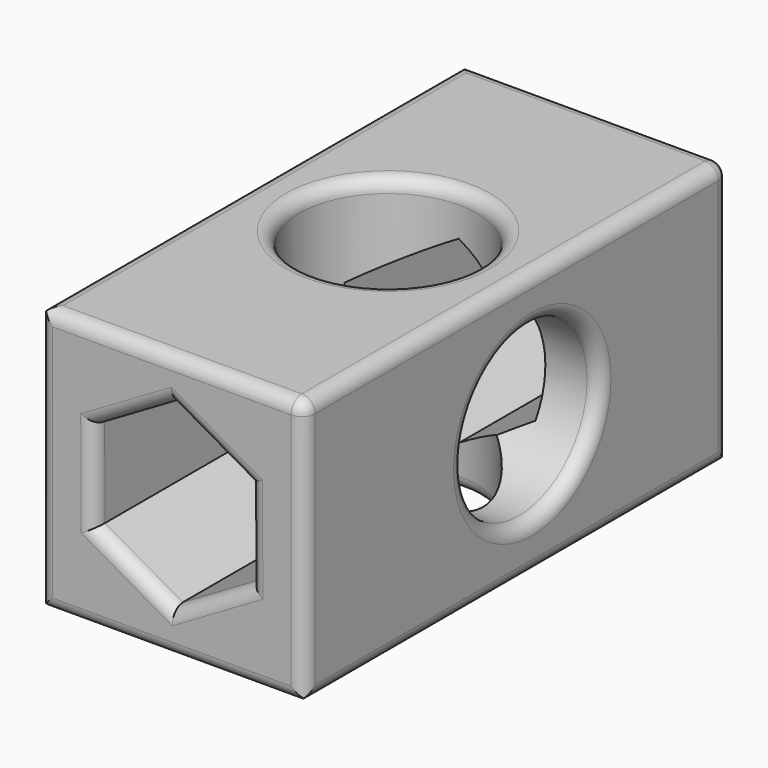
from build123d import *

# Parameters (mm, degrees)
F0_W           = 100
F0_H           = 100
F1_DEPTH       = 200
F2_DEPTH       = 25
F3_R           = 27.377441892
F4_DEPTH       = 67
F5_R           = 33.5014212571
F6_DEPTH       = 100.001
F7_R           = 32.0841158334
F8_DEPTH       = 50.001
F9_R           = 5
F10_T1_DEPTH   = 120
F10_T3_DEPTH   = 120
F10_T8_DEPTH   = 58.784451779
F10_T14_DEPTH  = 58.784451779
F10_T20_DEPTH  = 58.784451779
F10_T26_DEPTH  = 58.784451779
F10_T32_DEPTH  = 58.784451779
F10_T38_DEPTH  = 58.784451779
F10_T45_DEPTH  = 58.784451779
F10_T49_DEPTH  = 58.784451779
F10_T56_DEPTH  = 58.784451779
F10_T60_DEPTH  = 58.784451779
F10_T67_DEPTH  = 58.784451779
F10_T71_DEPTH  = 58.784451779
F10_T78_DEPTH  = 58.784451779
F10_T82_DEPTH  = 58.784451779
F10_T89_DEPTH  = 58.784451779
F10_T93_DEPTH  = 58.784451779
F10_T100_DEPTH = 58.784451779
F10_T104_DEPTH = 58.784451779
F11_T1_DEPTH   = 220.0048285071
F11_T3_DEPTH   = 120.0048285071
F12_T1_DEPTH   = 113.8468181408
F12_T3_DEPTH   = 115.0622872397
F12_T8_DEPTH   = 58.784451779
F12_T14_DEPTH  = 58.784451779
F12_T20_DEPTH  = 58.784451779
F12_T26_DEPTH  = 58.784451779
F12_T32_DEPTH  = 58.784451779
F12_T38_DEPTH  = 58.784451779
F12_T45_DEPTH  = 58.784451779
F12_T49_DEPTH  = 58.784451779
F12_T56_DEPTH  = 58.784451779
F12_T60_DEPTH  = 58.784451779
F12_T67_DEPTH  = 58.784451779
F12_T71_DEPTH  = 58.784451779
F12_T78_DEPTH  = 58.784451779
F12_T82_DEPTH  = 58.784451779
F12_T89_DEPTH  = 58.784451779
F12_T93_DEPTH  = 58.784451779
F12_T100_DEPTH = 58.784451779
F12_T104_DEPTH = 58.784451779


# Not quite as in the source:
# - a fillet or chamfer that OpenCascade refuses, or shapes differently, is made with other operations: its cross-section is extruded or revolved along the edge and cut away or added


with BuildPart() as f1:
    # F0 (on Front) → F1 (new body)
    with BuildSketch(Plane.XZ):
        Rectangle(F0_W, F0_H)
        Polygon((-29.3331185014, 16.7617821544), (-0.1504300923, 33.7841168716), (29.1826884091, 17.0223347172), (29.3331185014, -16.7617821544), (0.1504300923, -33.7841168716), (-29.1826884091, -17.0223347172), align=None, mode=Mode.SUBTRACT)
    extrude(amount=F1_DEPTH)

    # F0 (on Front) → F2 (join)
    with BuildSketch(Plane.XZ):
        Rectangle(F0_W, F0_H)
        Polygon((-29.3331185014, 16.7617821544), (-0.1504300923, 33.7841168716), (29.1826884091, 17.0223347172), (29.3331185014, -16.7617821544), (0.1504300923, -33.7841168716), (-29.1826884091, -17.0223347172), align=None, mode=Mode.SUBTRACT)
    extrude(amount=F2_DEPTH)

    # F3 (on Top) → F4 (cut)
    with BuildSketch(Plane.XY):
        with Locations((2.3286284413, -101.0887101293)):
            Circle(F3_R)
    extrude(amount=-F4_DEPTH, mode=Mode.SUBTRACT)

    # F5 (on face) → F6 (cut, through all)
    with BuildSketch(Plane.XY.offset(50)):
        with Locations((0, -98.0947613716)):
            Circle(F5_R)
    extrude(amount=-F6_DEPTH, mode=Mode.SUBTRACT)

    # F7 (on Right) → F8 (cut, through all)
    with BuildSketch(Plane.YZ):
        with Locations((-92.6209688187, 0)):
            Circle(F7_R)
    extrude(amount=F8_DEPTH, mode=Mode.SUBTRACT)

    # F9
    f9_edges = [f1.edges().sort_by_distance(p)[0] for p in [
        (0, 0, 50),
        (50, -100, 50),
        (-50, -100, 50),
        (0, -200, 50),
        (-33.501421, -98.094761, 50),
        (50, 0, 0),
        (50, -100, -50),
        (50, -200, 0),
        (50, -124.705085, 0),
    ]]
    fillet(f9_edges, radius=F9_R)

    # F10: fillet of radius 5 on 10 edges, made by hand

    # F10_s2 → F10_t1 (cut)
    with BuildSketch(Plane.XY.offset(-62.5)):
        with BuildLine():
            ThreePointArc((-45, -200), (-48.5355339059, -198.5355339059), (-50, -195))
            Line((-50, -195), (-50, -200))
            Line((-50, -200), (-45, -200))
        make_face()
    extrude(amount=F10_T1_DEPTH, mode=Mode.SUBTRACT)

    # F10_s4 → F10_t3 (cut)
    with BuildSketch(Plane.YZ.offset(-62.5)):
        with BuildLine():
            ThreePointArc((-200, -45), (-198.5355339059, -48.5355339059), (-195, -50))
            Line((-195, -50), (-200, -50))
            Line((-200, -50), (-200, -45))
        make_face()
    extrude(amount=F10_T3_DEPTH, mode=Mode.SUBTRACT)


with BuildPart() as f10_tool6:
    # F10_s7 → F10_t8 (new body)
    with BuildSketch(Plane(origin=(0.1308730798, 0, -29.3919345225), x_dir=(0, 1, 0), z_dir=(-0.0044526427, 0, 0.9999900869))):
        with BuildLine():
            ThreePointArc((-200, 34.2581934936), (-198.5355339059, 30.7226595876), (-195, 29.2581934936))
            Line((-195, 29.2581934936), (-200, 29.2581934936))
            Line((-200, 29.2581934936), (-200, 34.2581934936))
        make_face()
    extrude(amount=F10_T8_DEPTH)

    split(bisect_by=Plane(origin=(-14.7417742968, 0, 25.272949513), x_dir=(0, 1, 0), z_dir=(0.5038511452, 0, -0.8637904975)), keep=Keep.TOP)

    split(bisect_by=Plane(origin=(-14.5161291584, 0, -25.4032257944), x_dir=(0, 1, 0), z_dir=(0.4961389418, 0, 0.8682431402)), keep=Keep.TOP)


with BuildPart() as f1_1:
    add(f1.part)

    # F10_t5: cut F10_tool6
    add(f10_tool6.part, mode=Mode.SUBTRACT)


with BuildPart() as f10_tool12:
    # F10_s13 → F10_t14 (new body)
    with BuildSketch(Plane(origin=(-25.388725423, 0, -14.809306673), x_dir=(0, 1, 0), z_dir=(0.8637904975, 0, 0.5038511452))):
        with BuildLine():
            ThreePointArc((-200, 34.2581934936), (-198.5355339059, 30.7226595876), (-195, 29.2581934936))
            Line((-195, 29.2581934936), (-200, 29.2581934936))
            Line((-200, 29.2581934936), (-200, 34.2581934936))
        make_face()
    extrude(amount=F10_T14_DEPTH)

    split(bisect_by=Plane(origin=(-29.2579034553, 0, -0.1302762814), x_dir=(0, 1, 0), z_dir=(0.9999900869, 0, 0.0044526427)), keep=Keep.TOP)

    split(bisect_by=Plane(origin=(14.5161291584, 0, 25.4032257944), x_dir=(0, 1, 0), z_dir=(-0.4961389418, 0, -0.8682431402)), keep=Keep.TOP)


with BuildPart() as f1_2:
    add(f1_1.part)

    # F10_t11: cut F10_tool12
    add(f10_tool12.part, mode=Mode.SUBTRACT)


with BuildPart() as f10_tool18:
    # F10_s19 → F10_t20 (new body)
    with BuildSketch(Plane(origin=(-25.5195985028, 0, 14.5826278495), x_dir=(0, 1, 0), z_dir=(0.8682431402, 0, -0.4961389418))):
        with BuildLine():
            ThreePointArc((-200, 34.2581934936), (-198.5355339059, 30.7226595876), (-195, 29.2581934936))
            Line((-195, 29.2581934936), (-200, 29.2581934936))
            Line((-200, 29.2581934936), (-200, 34.2581934936))
        make_face()
    extrude(amount=F10_T20_DEPTH)

    split(bisect_by=Plane(origin=(-14.7417742968, 0, 25.272949513), x_dir=(0, 1, 0), z_dir=(0.5038511452, 0, -0.8637904975)), keep=Keep.TOP)

    split(bisect_by=Plane(origin=(29.2579034553, 0, 0.1302762814), x_dir=(0, 1, 0), z_dir=(-0.9999900869, 0, -0.0044526427)), keep=Keep.TOP)


with BuildPart() as f1_3:
    add(f1_2.part)

    # F10_t17: cut F10_tool18
    add(f10_tool18.part, mode=Mode.SUBTRACT)


with BuildPart() as f10_tool24:
    # F10_s25 → F10_t26 (new body)
    with BuildSketch(Plane(origin=(-0.1308730798, 0, 29.3919345225), x_dir=(0, 1, 0), z_dir=(0.0044526427, 0, -0.9999900869))):
        with BuildLine():
            ThreePointArc((-200, 34.2581934936), (-198.5355339059, 30.7226595876), (-195, 29.2581934936))
            Line((-195, 29.2581934936), (-200, 29.2581934936))
            Line((-200, 29.2581934936), (-200, 34.2581934936))
        make_face()
    extrude(amount=F10_T26_DEPTH)

    split(bisect_by=Plane(origin=(14.5161291584, 0, 25.4032257944), x_dir=(0, 1, 0), z_dir=(-0.4961389418, 0, -0.8682431402)), keep=Keep.TOP)

    split(bisect_by=Plane(origin=(14.7417742968, 0, -25.272949513), x_dir=(0, 1, 0), z_dir=(-0.5038511452, 0, 0.8637904975)), keep=Keep.TOP)


with BuildPart() as f1_4:
    add(f1_3.part)

    # F10_t23: cut F10_tool24
    add(f10_tool24.part, mode=Mode.SUBTRACT)


with BuildPart() as f10_tool30:
    # F10_s31 → F10_t32 (new body)
    with BuildSketch(Plane(origin=(25.388725423, 0, 14.809306673), x_dir=(0, 1, 0), z_dir=(-0.8637904975, 0, -0.5038511452))):
        with BuildLine():
            ThreePointArc((-200, 34.2581934936), (-198.5355339059, 30.7226595876), (-195, 29.2581934936))
            Line((-195, 29.2581934936), (-200, 29.2581934936))
            Line((-200, 29.2581934936), (-200, 34.2581934936))
        make_face()
    extrude(amount=F10_T32_DEPTH)

    split(bisect_by=Plane(origin=(29.2579034553, 0, 0.1302762814), x_dir=(0, 1, 0), z_dir=(-0.9999900869, 0, -0.0044526427)), keep=Keep.TOP)

    split(bisect_by=Plane(origin=(-14.5161291584, 0, -25.4032257944), x_dir=(0, 1, 0), z_dir=(0.4961389418, 0, 0.8682431402)), keep=Keep.TOP)


with BuildPart() as f1_5:
    add(f1_4.part)

    # F10_t29: cut F10_tool30
    add(f10_tool30.part, mode=Mode.SUBTRACT)


with BuildPart() as f10_tool36:
    # F10_s37 → F10_t38 (new body)
    with BuildSketch(Plane(origin=(25.5195985028, 0, -14.5826278495), x_dir=(0, 1, 0), z_dir=(-0.8682431402, 0, 0.4961389418))):
        with BuildLine():
            ThreePointArc((-200, 34.2581934936), (-198.5355339059, 30.7226595876), (-195, 29.2581934936))
            Line((-195, 29.2581934936), (-200, 29.2581934936))
            Line((-200, 29.2581934936), (-200, 34.2581934936))
        make_face()
    extrude(amount=F10_T38_DEPTH)

    split(bisect_by=Plane(origin=(-29.2579034553, 0, -0.1302762814), x_dir=(0, 1, 0), z_dir=(0.9999900869, 0, 0.0044526427)), keep=Keep.TOP)

    split(bisect_by=Plane(origin=(14.7417742968, 0, -25.272949513), x_dir=(0, 1, 0), z_dir=(-0.5038511452, 0, 0.8637904975)), keep=Keep.TOP)


with BuildPart() as f1_6:
    add(f1_5.part)

    # F10_t35: cut F10_tool36
    add(f10_tool36.part, mode=Mode.SUBTRACT)


with BuildPart() as f10_tool43:
    # F10_s44 → F10_t45 (new body)
    with BuildSketch(Plane(origin=(0.1308730798, 0, -29.3919345225), x_dir=(0, 1, 0), z_dir=(-0.0044526427, 0, 0.9999900869))):
        with BuildLine():
            ThreePointArc((-200, 34.2581934936), (-198.5355339059, 30.7226595876), (-195, 29.2581934936))
            Line((-195, 29.2581934936), (-200, 29.2581934936))
            Line((-200, 29.2581934936), (-200, 34.2581934936))
        make_face()
    extrude(amount=F10_T45_DEPTH)

    split(bisect_by=Plane(origin=(-14.5161291584, 0, -25.4032257944), x_dir=(0, 1, 0), z_dir=(-0.4961389418, 0, -0.8682431402)), keep=Keep.TOP)


with BuildPart() as f10_tool47:
    # F10_s48 → F10_t49 (new body)
    with BuildSketch(Plane(origin=(25.5195985028, 0, -14.5826278495), x_dir=(0, 1, 0), z_dir=(-0.8682431402, 0, 0.4961389418))):
        with BuildLine():
            ThreePointArc((-200, 34.2581934936), (-198.5355339059, 30.7226595876), (-195, 29.2581934936))
            Line((-195, 29.2581934936), (-200, 29.2581934936))
            Line((-200, 29.2581934936), (-200, 34.2581934936))
        make_face()
    extrude(amount=F10_T49_DEPTH)

    split(bisect_by=Plane(origin=(-29.2579034553, 0, -0.1302762814), x_dir=(0, 1, 0), z_dir=(-0.9999900869, 0, -0.0044526427)), keep=Keep.TOP)


with BuildPart() as f10_tool43_1:
    add(f10_tool43.part)

    # F10_t51: intersect F10_tool47
    add(f10_tool47.part, mode=Mode.INTERSECT)


with BuildPart() as f1_7:
    add(f1_6.part)

    # F10_t41: cut F10_tool43
    add(f10_tool43_1.part, mode=Mode.SUBTRACT)


with BuildPart() as f10_tool54:
    # F10_s55 → F10_t56 (new body)
    with BuildSketch(Plane(origin=(0.1308730798, 0, -29.3919345225), x_dir=(0, 1, 0), z_dir=(-0.0044526427, 0, 0.9999900869))):
        with BuildLine():
            ThreePointArc((-200, 34.2581934936), (-198.5355339059, 30.7226595876), (-195, 29.2581934936))
            Line((-195, 29.2581934936), (-200, 29.2581934936))
            Line((-200, 29.2581934936), (-200, 34.2581934936))
        make_face()
    extrude(amount=F10_T56_DEPTH)

    split(bisect_by=Plane(origin=(-14.7417742968, 0, 25.272949513), x_dir=(0, 1, 0), z_dir=(-0.5038511452, 0, 0.8637904975)), keep=Keep.TOP)


with BuildPart() as f10_tool58:
    # F10_s59 → F10_t60 (new body)
    with BuildSketch(Plane(origin=(-25.388725423, 0, -14.809306673), x_dir=(0, 1, 0), z_dir=(0.8637904975, 0, 0.5038511452))):
        with BuildLine():
            ThreePointArc((-200, 34.2581934936), (-198.5355339059, 30.7226595876), (-195, 29.2581934936))
            Line((-195, 29.2581934936), (-200, 29.2581934936))
            Line((-200, 29.2581934936), (-200, 34.2581934936))
        make_face()
    extrude(amount=F10_T60_DEPTH)

    split(bisect_by=Plane(origin=(-29.2579034553, 0, -0.1302762814), x_dir=(0, 1, 0), z_dir=(-0.9999900869, 0, -0.0044526427)), keep=Keep.TOP)


with BuildPart() as f10_tool54_1:
    add(f10_tool54.part)

    # F10_t62: intersect F10_tool58
    add(f10_tool58.part, mode=Mode.INTERSECT)


with BuildPart() as f1_8:
    add(f1_7.part)

    # F10_t52: cut F10_tool54
    add(f10_tool54_1.part, mode=Mode.SUBTRACT)


with BuildPart() as f10_tool65:
    # F10_s66 → F10_t67 (new body)
    with BuildSketch(Plane(origin=(-25.388725423, 0, -14.809306673), x_dir=(0, 1, 0), z_dir=(0.8637904975, 0, 0.5038511452))):
        with BuildLine():
            ThreePointArc((-200, 34.2581934936), (-198.5355339059, 30.7226595876), (-195, 29.2581934936))
            Line((-195, 29.2581934936), (-200, 29.2581934936))
            Line((-200, 29.2581934936), (-200, 34.2581934936))
        make_face()
    extrude(amount=F10_T67_DEPTH)

    split(bisect_by=Plane(origin=(14.5161291584, 0, 25.4032257944), x_dir=(0, 1, 0), z_dir=(0.4961389418, 0, 0.8682431402)), keep=Keep.TOP)


with BuildPart() as f10_tool69:
    # F10_s70 → F10_t71 (new body)
    with BuildSketch(Plane(origin=(-25.5195985028, 0, 14.5826278495), x_dir=(0, 1, 0), z_dir=(0.8682431402, 0, -0.4961389418))):
        with BuildLine():
            ThreePointArc((-200, 34.2581934936), (-198.5355339059, 30.7226595876), (-195, 29.2581934936))
            Line((-195, 29.2581934936), (-200, 29.2581934936))
            Line((-200, 29.2581934936), (-200, 34.2581934936))
        make_face()
    extrude(amount=F10_T71_DEPTH)

    split(bisect_by=Plane(origin=(-14.7417742968, 0, 25.272949513), x_dir=(0, 1, 0), z_dir=(-0.5038511452, 0, 0.8637904975)), keep=Keep.TOP)


with BuildPart() as f10_tool65_1:
    add(f10_tool65.part)

    # F10_t73: intersect F10_tool69
    add(f10_tool69.part, mode=Mode.INTERSECT)


with BuildPart() as f1_9:
    add(f1_8.part)

    # F10_t63: cut F10_tool65
    add(f10_tool65_1.part, mode=Mode.SUBTRACT)


with BuildPart() as f10_tool76:
    # F10_s77 → F10_t78 (new body)
    with BuildSketch(Plane(origin=(-25.5195985028, 0, 14.5826278495), x_dir=(0, 1, 0), z_dir=(0.8682431402, 0, -0.4961389418))):
        with BuildLine():
            ThreePointArc((-200, 34.2581934936), (-198.5355339059, 30.7226595876), (-195, 29.2581934936))
            Line((-195, 29.2581934936), (-200, 29.2581934936))
            Line((-200, 29.2581934936), (-200, 34.2581934936))
        make_face()
    extrude(amount=F10_T78_DEPTH)

    split(bisect_by=Plane(origin=(29.2579034553, 0, 0.1302762814), x_dir=(0, 1, 0), z_dir=(0.9999900869, 0, 0.0044526427)), keep=Keep.TOP)


with BuildPart() as f10_tool80:
    # F10_s81 → F10_t82 (new body)
    with BuildSketch(Plane(origin=(-0.1308730798, 0, 29.3919345225), x_dir=(0, 1, 0), z_dir=(0.0044526427, 0, -0.9999900869))):
        with BuildLine():
            ThreePointArc((-200, 34.2581934936), (-198.5355339059, 30.7226595876), (-195, 29.2581934936))
            Line((-195, 29.2581934936), (-200, 29.2581934936))
            Line((-200, 29.2581934936), (-200, 34.2581934936))
        make_face()
    extrude(amount=F10_T82_DEPTH)

    split(bisect_by=Plane(origin=(14.5161291584, 0, 25.4032257944), x_dir=(0, 1, 0), z_dir=(0.4961389418, 0, 0.8682431402)), keep=Keep.TOP)


with BuildPart() as f10_tool76_1:
    add(f10_tool76.part)

    # F10_t84: intersect F10_tool80
    add(f10_tool80.part, mode=Mode.INTERSECT)


with BuildPart() as f1_10:
    add(f1_9.part)

    # F10_t74: cut F10_tool76
    add(f10_tool76_1.part, mode=Mode.SUBTRACT)


with BuildPart() as f10_tool87:
    # F10_s88 → F10_t89 (new body)
    with BuildSketch(Plane(origin=(-0.1308730798, 0, 29.3919345225), x_dir=(0, 1, 0), z_dir=(0.0044526427, 0, -0.9999900869))):
        with BuildLine():
            ThreePointArc((-200, 34.2581934936), (-198.5355339059, 30.7226595876), (-195, 29.2581934936))
            Line((-195, 29.2581934936), (-200, 29.2581934936))
            Line((-200, 29.2581934936), (-200, 34.2581934936))
        make_face()
    extrude(amount=F10_T89_DEPTH)

    split(bisect_by=Plane(origin=(14.7417742968, 0, -25.272949513), x_dir=(0, 1, 0), z_dir=(0.5038511452, 0, -0.8637904975)), keep=Keep.TOP)


with BuildPart() as f10_tool91:
    # F10_s92 → F10_t93 (new body)
    with BuildSketch(Plane(origin=(25.388725423, 0, 14.809306673), x_dir=(0, 1, 0), z_dir=(-0.8637904975, 0, -0.5038511452))):
        with BuildLine():
            ThreePointArc((-200, 34.2581934936), (-198.5355339059, 30.7226595876), (-195, 29.2581934936))
            Line((-195, 29.2581934936), (-200, 29.2581934936))
            Line((-200, 29.2581934936), (-200, 34.2581934936))
        make_face()
    extrude(amount=F10_T93_DEPTH)

    split(bisect_by=Plane(origin=(29.2579034553, 0, 0.1302762814), x_dir=(0, 1, 0), z_dir=(0.9999900869, 0, 0.0044526427)), keep=Keep.TOP)


with BuildPart() as f10_tool87_1:
    add(f10_tool87.part)

    # F10_t95: intersect F10_tool91
    add(f10_tool91.part, mode=Mode.INTERSECT)


with BuildPart() as f1_11:
    add(f1_10.part)

    # F10_t85: cut F10_tool87
    add(f10_tool87_1.part, mode=Mode.SUBTRACT)


with BuildPart() as f10_tool98:
    # F10_s99 → F10_t100 (new body)
    with BuildSketch(Plane(origin=(25.388725423, 0, 14.809306673), x_dir=(0, 1, 0), z_dir=(-0.8637904975, 0, -0.5038511452))):
        with BuildLine():
            ThreePointArc((-200, 34.2581934936), (-198.5355339059, 30.7226595876), (-195, 29.2581934936))
            Line((-195, 29.2581934936), (-200, 29.2581934936))
            Line((-200, 29.2581934936), (-200, 34.2581934936))
        make_face()
    extrude(amount=F10_T100_DEPTH)

    split(bisect_by=Plane(origin=(-14.5161291584, 0, -25.4032257944), x_dir=(0, 1, 0), z_dir=(-0.4961389418, 0, -0.8682431402)), keep=Keep.TOP)


with BuildPart() as f10_tool102:
    # F10_s103 → F10_t104 (new body)
    with BuildSketch(Plane(origin=(25.5195985028, 0, -14.5826278495), x_dir=(0, 1, 0), z_dir=(-0.8682431402, 0, 0.4961389418))):
        with BuildLine():
            ThreePointArc((-200, 34.2581934936), (-198.5355339059, 30.7226595876), (-195, 29.2581934936))
            Line((-195, 29.2581934936), (-200, 29.2581934936))
            Line((-200, 29.2581934936), (-200, 34.2581934936))
        make_face()
    extrude(amount=F10_T104_DEPTH)

    split(bisect_by=Plane(origin=(14.7417742968, 0, -25.272949513), x_dir=(0, 1, 0), z_dir=(0.5038511452, 0, -0.8637904975)), keep=Keep.TOP)


with BuildPart() as f10_tool98_1:
    add(f10_tool98.part)

    # F10_t106: intersect F10_tool102
    add(f10_tool102.part, mode=Mode.INTERSECT)


with BuildPart() as f1_12:
    add(f1_11.part)

    # F10_t96: cut F10_tool98
    add(f10_tool98_1.part, mode=Mode.SUBTRACT)

    # F11: fillet of radius 5 on 5 edges, made by hand

    # F11_s2 → F11_t1 (cut)
    with BuildSketch(Plane.XZ.offset(-12.5024142536)):
        with BuildLine():
            ThreePointArc((-44.9990343146, -50.0004), (-48.5355339059, -48.5355339059), (-50.0004, -44.9990343146))
            Line((-50.0004, -44.9990343146), (-50.5005365685, -44.9990343146))
            ThreePointArc((-50.5005365685, -44.9990343146), (-50.5001365685, -47.4995171573), (-50.5001365685, -50))
            Line((-50.5001365685, -50), (-50, -50.5001365685))
            ThreePointArc((-50, -50.5001365685), (-47.4995171573, -50.5001365685), (-44.9990343146, -50.5005365685))
            Line((-44.9990343146, -50.5005365685), (-44.9990343146, -50.0004))
        make_face()
    extrude(amount=F11_T1_DEPTH, mode=Mode.SUBTRACT)

    # F11_s4 → F11_t3 (cut)
    with BuildSketch(Plane.YZ.offset(-62.5024142536)):
        with BuildLine():
            ThreePointArc((-5.0009656854, -50.0004), (-1.4644660941, -48.5355339059), (0.0004, -44.9990343146))
            Line((0.0004, -44.9990343146), (0.5005365685, -44.9990343146))
            ThreePointArc((0.5005365685, -44.9990343146), (0.5001365685, -47.4995171573), (0.5001365685, -50))
            Line((0.5001365685, -50), (0, -50.5001365685))
            ThreePointArc((0, -50.5001365685), (-2.5004828427, -50.5001365685), (-5.0009656854, -50.5005365685))
            Line((-5.0009656854, -50.5005365685), (-5.0009656854, -50.0004))
        make_face()
    extrude(amount=F11_T3_DEPTH, mode=Mode.SUBTRACT)

    # F11_s5 → F11_t6 (revolve, cut)
    with BuildSketch(Plane.XZ.offset(98.0947613716)):
        with BuildLine():
            ThreePointArc((38.5023869425, -50.0004), (34.9658873512, -48.5355339059), (33.5010212571, -44.9990343146))
            Line((33.5010212571, -44.9990343146), (33.0008846886, -44.9990343146))
            ThreePointArc((33.0008846886, -44.9990343146), (33.0012846886, -47.4995171573), (33.0012846886, -50))
            Line((33.0012846886, -50), (33.5014212571, -50.5001365685))
            ThreePointArc((33.5014212571, -50.5001365685), (36.0019040998, -50.5001365685), (38.5023869425, -50.5005365685))
            Line((38.5023869425, -50.5005365685), (38.5023869425, -50.0004))
        make_face()
    revolve(axis=Axis((0, -98.0947613716, -50), (0, 0, 1)), mode=Mode.SUBTRACT)

    # F12: fillet of radius 5 on 10 edges, made by hand

    # F12_s2 → F12_t1 (cut)
    with BuildSketch(Plane.YZ.offset(-59.4234090704)):
        with BuildLine():
            ThreePointArc((0, -44.9999999999), (-0.380602305, -46.9134170835), (-1.4644659742, -48.535533786))
            ThreePointArc((-1.4644659742, -48.535533786), (-0.3925018153, -46.9421553804), (0, -45.0622872397))
            Line((0, -45.0622872397), (0, -44.9999999999))
        make_face()
    extrude(amount=F12_T1_DEPTH, mode=Mode.SUBTRACT)

    # F12_s4 → F12_t3 (cut)
    with BuildSketch(Plane.XY.offset(-57.5622872397)):
        with BuildLine():
            ThreePointArc((-45, 0), (-48.5355339059, -1.4644660941), (-50, -5))
            Line((-50, -5), (-50, 0))
            Line((-50, 0), (-45, 0))
        make_face()
    extrude(amount=F12_T3_DEPTH, mode=Mode.SUBTRACT)


with BuildPart() as f12_tool6:
    # F12_s7 → F12_t8 (new body)
    with BuildSketch(Plane(origin=(0.1308730798, 0, -29.3919345225), x_dir=(0, 1, 0), z_dir=(-0.0044526427, 0, 0.9999900869))):
        with BuildLine():
            ThreePointArc((0, 34.2581934936), (-1.4644660941, 30.7226595876), (-5, 29.2581934936))
            Line((-5, 29.2581934936), (0, 29.2581934936))
            Line((0, 29.2581934936), (0, 34.2581934936))
        make_face()
    extrude(amount=F12_T8_DEPTH)

    split(bisect_by=Plane(origin=(-14.5161291584, 0, -25.4032257944), x_dir=(0, 1, 0), z_dir=(0.4961389418, 0, 0.8682431402)), keep=Keep.TOP)

    split(bisect_by=Plane(origin=(-14.7417742968, 0, 25.272949513), x_dir=(0, 1, 0), z_dir=(0.5038511452, 0, -0.8637904975)), keep=Keep.TOP)


with BuildPart() as f1_13:
    add(f1_12.part)

    # F12_t5: cut F12_tool6
    add(f12_tool6.part, mode=Mode.SUBTRACT)


with BuildPart() as f12_tool12:
    # F12_s13 → F12_t14 (new body)
    with BuildSketch(Plane(origin=(25.5195985028, 0, -14.5826278495), x_dir=(0, 1, 0), z_dir=(-0.8682431402, 0, 0.4961389418))):
        with BuildLine():
            ThreePointArc((0, 34.2581934936), (-1.4644660941, 30.7226595876), (-5, 29.2581934936))
            Line((-5, 29.2581934936), (0, 29.2581934936))
            Line((0, 29.2581934936), (0, 34.2581934936))
        make_face()
    extrude(amount=F12_T14_DEPTH)

    split(bisect_by=Plane(origin=(-29.2579034553, 0, -0.1302762814), x_dir=(0, 1, 0), z_dir=(0.9999900869, 0, 0.0044526427)), keep=Keep.TOP)

    split(bisect_by=Plane(origin=(14.7417742968, 0, -25.272949513), x_dir=(0, 1, 0), z_dir=(-0.5038511452, 0, 0.8637904975)), keep=Keep.TOP)


with BuildPart() as f1_14:
    add(f1_13.part)

    # F12_t11: cut F12_tool12
    add(f12_tool12.part, mode=Mode.SUBTRACT)


with BuildPart() as f12_tool18:
    # F12_s19 → F12_t20 (new body)
    with BuildSketch(Plane(origin=(-25.388725423, 0, -14.809306673), x_dir=(0, 1, 0), z_dir=(0.8637904975, 0, 0.5038511452))):
        with BuildLine():
            ThreePointArc((0, 34.2581934936), (-1.4644660941, 30.7226595876), (-5, 29.2581934936))
            Line((-5, 29.2581934936), (0, 29.2581934936))
            Line((0, 29.2581934936), (0, 34.2581934936))
        make_face()
    extrude(amount=F12_T20_DEPTH)

    split(bisect_by=Plane(origin=(-29.2579034553, 0, -0.1302762814), x_dir=(0, 1, 0), z_dir=(0.9999900869, 0, 0.0044526427)), keep=Keep.TOP)

    split(bisect_by=Plane(origin=(14.5161291584, 0, 25.4032257944), x_dir=(0, 1, 0), z_dir=(-0.4961389418, 0, -0.8682431402)), keep=Keep.TOP)


with BuildPart() as f1_15:
    add(f1_14.part)

    # F12_t17: cut F12_tool18
    add(f12_tool18.part, mode=Mode.SUBTRACT)


with BuildPart() as f12_tool24:
    # F12_s25 → F12_t26 (new body)
    with BuildSketch(Plane(origin=(25.388725423, 0, 14.809306673), x_dir=(0, 1, 0), z_dir=(-0.8637904975, 0, -0.5038511452))):
        with BuildLine():
            ThreePointArc((0, 34.2581934936), (-1.4644660941, 30.7226595876), (-5, 29.2581934936))
            Line((-5, 29.2581934936), (0, 29.2581934936))
            Line((0, 29.2581934936), (0, 34.2581934936))
        make_face()
    extrude(amount=F12_T26_DEPTH)

    split(bisect_by=Plane(origin=(-14.5161291584, 0, -25.4032257944), x_dir=(0, 1, 0), z_dir=(0.4961389418, 0, 0.8682431402)), keep=Keep.TOP)

    split(bisect_by=Plane(origin=(29.2579034553, 0, 0.1302762814), x_dir=(0, 1, 0), z_dir=(-0.9999900869, 0, -0.0044526427)), keep=Keep.TOP)


with BuildPart() as f1_16:
    add(f1_15.part)

    # F12_t23: cut F12_tool24
    add(f12_tool24.part, mode=Mode.SUBTRACT)


with BuildPart() as f12_tool30:
    # F12_s31 → F12_t32 (new body)
    with BuildSketch(Plane(origin=(-25.5195985028, 0, 14.5826278495), x_dir=(0, 1, 0), z_dir=(0.8682431402, 0, -0.4961389418))):
        with BuildLine():
            ThreePointArc((0, 34.2581934936), (-1.4644660941, 30.7226595876), (-5, 29.2581934936))
            Line((-5, 29.2581934936), (0, 29.2581934936))
            Line((0, 29.2581934936), (0, 34.2581934936))
        make_face()
    extrude(amount=F12_T32_DEPTH)

    split(bisect_by=Plane(origin=(-14.7417742968, 0, 25.272949513), x_dir=(0, 1, 0), z_dir=(0.5038511452, 0, -0.8637904975)), keep=Keep.TOP)

    split(bisect_by=Plane(origin=(29.2579034553, 0, 0.1302762814), x_dir=(0, 1, 0), z_dir=(-0.9999900869, 0, -0.0044526427)), keep=Keep.TOP)


with BuildPart() as f1_17:
    add(f1_16.part)

    # F12_t29: cut F12_tool30
    add(f12_tool30.part, mode=Mode.SUBTRACT)


with BuildPart() as f12_tool36:
    # F12_s37 → F12_t38 (new body)
    with BuildSketch(Plane(origin=(-0.1308730798, 0, 29.3919345225), x_dir=(0, 1, 0), z_dir=(0.0044526427, 0, -0.9999900869))):
        with BuildLine():
            ThreePointArc((0, 34.2581934936), (-1.4644660941, 30.7226595876), (-5, 29.2581934936))
            Line((-5, 29.2581934936), (0, 29.2581934936))
            Line((0, 29.2581934936), (0, 34.2581934936))
        make_face()
    extrude(amount=F12_T38_DEPTH)

    split(bisect_by=Plane(origin=(14.7417742968, 0, -25.272949513), x_dir=(0, 1, 0), z_dir=(-0.5038511452, 0, 0.8637904975)), keep=Keep.TOP)

    split(bisect_by=Plane(origin=(14.5161291584, 0, 25.4032257944), x_dir=(0, 1, 0), z_dir=(-0.4961389418, 0, -0.8682431402)), keep=Keep.TOP)


with BuildPart() as f1_18:
    add(f1_17.part)

    # F12_t35: cut F12_tool36
    add(f12_tool36.part, mode=Mode.SUBTRACT)


with BuildPart() as f12_tool43:
    # F12_s44 → F12_t45 (new body)
    with BuildSketch(Plane(origin=(0.1308730798, 0, -29.3919345225), x_dir=(0, 1, 0), z_dir=(-0.0044526427, 0, 0.9999900869))):
        with BuildLine():
            ThreePointArc((0, 34.2581934936), (-1.4644660941, 30.7226595876), (-5, 29.2581934936))
            Line((-5, 29.2581934936), (0, 29.2581934936))
            Line((0, 29.2581934936), (0, 34.2581934936))
        make_face()
    extrude(amount=F12_T45_DEPTH)

    split(bisect_by=Plane(origin=(-14.5161291584, 0, -25.4032257944), x_dir=(0, 1, 0), z_dir=(-0.4961389418, 0, -0.8682431402)), keep=Keep.TOP)


with BuildPart() as f12_tool47:
    # F12_s48 → F12_t49 (new body)
    with BuildSketch(Plane(origin=(25.5195985028, 0, -14.5826278495), x_dir=(0, 1, 0), z_dir=(-0.8682431402, 0, 0.4961389418))):
        with BuildLine():
            ThreePointArc((0, 34.2581934936), (-1.4644660941, 30.7226595876), (-5, 29.2581934936))
            Line((-5, 29.2581934936), (0, 29.2581934936))
            Line((0, 29.2581934936), (0, 34.2581934936))
        make_face()
    extrude(amount=F12_T49_DEPTH)

    split(bisect_by=Plane(origin=(-29.2579034553, 0, -0.1302762814), x_dir=(0, 1, 0), z_dir=(-0.9999900869, 0, -0.0044526427)), keep=Keep.TOP)


with BuildPart() as f12_tool43_1:
    add(f12_tool43.part)

    # F12_t51: intersect F12_tool47
    add(f12_tool47.part, mode=Mode.INTERSECT)


with BuildPart() as f1_19:
    add(f1_18.part)

    # F12_t41: cut F12_tool43
    add(f12_tool43_1.part, mode=Mode.SUBTRACT)


with BuildPart() as f12_tool54:
    # F12_s55 → F12_t56 (new body)
    with BuildSketch(Plane(origin=(0.1308730798, 0, -29.3919345225), x_dir=(0, 1, 0), z_dir=(-0.0044526427, 0, 0.9999900869))):
        with BuildLine():
            ThreePointArc((0, 34.2581934936), (-1.4644660941, 30.7226595876), (-5, 29.2581934936))
            Line((-5, 29.2581934936), (0, 29.2581934936))
            Line((0, 29.2581934936), (0, 34.2581934936))
        make_face()
    extrude(amount=F12_T56_DEPTH)

    split(bisect_by=Plane(origin=(-14.7417742968, 0, 25.272949513), x_dir=(0, 1, 0), z_dir=(-0.5038511452, 0, 0.8637904975)), keep=Keep.TOP)


with BuildPart() as f12_tool58:
    # F12_s59 → F12_t60 (new body)
    with BuildSketch(Plane(origin=(-25.388725423, 0, -14.809306673), x_dir=(0, 1, 0), z_dir=(0.8637904975, 0, 0.5038511452))):
        with BuildLine():
            ThreePointArc((0, 34.2581934936), (-1.4644660941, 30.7226595876), (-5, 29.2581934936))
            Line((-5, 29.2581934936), (0, 29.2581934936))
            Line((0, 29.2581934936), (0, 34.2581934936))
        make_face()
    extrude(amount=F12_T60_DEPTH)

    split(bisect_by=Plane(origin=(-29.2579034553, 0, -0.1302762814), x_dir=(0, 1, 0), z_dir=(-0.9999900869, 0, -0.0044526427)), keep=Keep.TOP)


with BuildPart() as f12_tool54_1:
    add(f12_tool54.part)

    # F12_t62: intersect F12_tool58
    add(f12_tool58.part, mode=Mode.INTERSECT)


with BuildPart() as f1_20:
    add(f1_19.part)

    # F12_t52: cut F12_tool54
    add(f12_tool54_1.part, mode=Mode.SUBTRACT)


with BuildPart() as f12_tool65:
    # F12_s66 → F12_t67 (new body)
    with BuildSketch(Plane(origin=(25.5195985028, 0, -14.5826278495), x_dir=(0, 1, 0), z_dir=(-0.8682431402, 0, 0.4961389418))):
        with BuildLine():
            ThreePointArc((0, 34.2581934936), (-1.4644660941, 30.7226595876), (-5, 29.2581934936))
            Line((-5, 29.2581934936), (0, 29.2581934936))
            Line((0, 29.2581934936), (0, 34.2581934936))
        make_face()
    extrude(amount=F12_T67_DEPTH)

    split(bisect_by=Plane(origin=(14.7417742968, 0, -25.272949513), x_dir=(0, 1, 0), z_dir=(0.5038511452, 0, -0.8637904975)), keep=Keep.TOP)


with BuildPart() as f12_tool69:
    # F12_s70 → F12_t71 (new body)
    with BuildSketch(Plane(origin=(25.388725423, 0, 14.809306673), x_dir=(0, 1, 0), z_dir=(-0.8637904975, 0, -0.5038511452))):
        with BuildLine():
            ThreePointArc((0, 34.2581934936), (-1.4644660941, 30.7226595876), (-5, 29.2581934936))
            Line((-5, 29.2581934936), (0, 29.2581934936))
            Line((0, 29.2581934936), (0, 34.2581934936))
        make_face()
    extrude(amount=F12_T71_DEPTH)

    split(bisect_by=Plane(origin=(-14.5161291584, 0, -25.4032257944), x_dir=(0, 1, 0), z_dir=(-0.4961389418, 0, -0.8682431402)), keep=Keep.TOP)


with BuildPart() as f12_tool65_1:
    add(f12_tool65.part)

    # F12_t73: intersect F12_tool69
    add(f12_tool69.part, mode=Mode.INTERSECT)


with BuildPart() as f1_21:
    add(f1_20.part)

    # F12_t63: cut F12_tool65
    add(f12_tool65_1.part, mode=Mode.SUBTRACT)


with BuildPart() as f12_tool76:
    # F12_s77 → F12_t78 (new body)
    with BuildSketch(Plane(origin=(-25.388725423, 0, -14.809306673), x_dir=(0, 1, 0), z_dir=(0.8637904975, 0, 0.5038511452))):
        with BuildLine():
            ThreePointArc((0, 34.2581934936), (-1.4644660941, 30.7226595876), (-5, 29.2581934936))
            Line((-5, 29.2581934936), (0, 29.2581934936))
            Line((0, 29.2581934936), (0, 34.2581934936))
        make_face()
    extrude(amount=F12_T78_DEPTH)

    split(bisect_by=Plane(origin=(14.5161291584, 0, 25.4032257944), x_dir=(0, 1, 0), z_dir=(0.4961389418, 0, 0.8682431402)), keep=Keep.TOP)


with BuildPart() as f12_tool80:
    # F12_s81 → F12_t82 (new body)
    with BuildSketch(Plane(origin=(-25.5195985028, 0, 14.5826278495), x_dir=(0, 1, 0), z_dir=(0.8682431402, 0, -0.4961389418))):
        with BuildLine():
            ThreePointArc((0, 34.2581934936), (-1.4644660941, 30.7226595876), (-5, 29.2581934936))
            Line((-5, 29.2581934936), (0, 29.2581934936))
            Line((0, 29.2581934936), (0, 34.2581934936))
        make_face()
    extrude(amount=F12_T82_DEPTH)

    split(bisect_by=Plane(origin=(-14.7417742968, 0, 25.272949513), x_dir=(0, 1, 0), z_dir=(-0.5038511452, 0, 0.8637904975)), keep=Keep.TOP)


with BuildPart() as f12_tool76_1:
    add(f12_tool76.part)

    # F12_t84: intersect F12_tool80
    add(f12_tool80.part, mode=Mode.INTERSECT)


with BuildPart() as f1_22:
    add(f1_21.part)

    # F12_t74: cut F12_tool76
    add(f12_tool76_1.part, mode=Mode.SUBTRACT)


with BuildPart() as f12_tool87:
    # F12_s88 → F12_t89 (new body)
    with BuildSketch(Plane(origin=(25.388725423, 0, 14.809306673), x_dir=(0, 1, 0), z_dir=(-0.8637904975, 0, -0.5038511452))):
        with BuildLine():
            ThreePointArc((0, 34.2581934936), (-1.4644660941, 30.7226595876), (-5, 29.2581934936))
            Line((-5, 29.2581934936), (0, 29.2581934936))
            Line((0, 29.2581934936), (0, 34.2581934936))
        make_face()
    extrude(amount=F12_T89_DEPTH)

    split(bisect_by=Plane(origin=(29.2579034553, 0, 0.1302762814), x_dir=(0, 1, 0), z_dir=(0.9999900869, 0, 0.0044526427)), keep=Keep.TOP)


with BuildPart() as f12_tool91:
    # F12_s92 → F12_t93 (new body)
    with BuildSketch(Plane(origin=(-0.1308730798, 0, 29.3919345225), x_dir=(0, 1, 0), z_dir=(0.0044526427, 0, -0.9999900869))):
        with BuildLine():
            ThreePointArc((0, 34.2581934936), (-1.4644660941, 30.7226595876), (-5, 29.2581934936))
            Line((-5, 29.2581934936), (0, 29.2581934936))
            Line((0, 29.2581934936), (0, 34.2581934936))
        make_face()
    extrude(amount=F12_T93_DEPTH)

    split(bisect_by=Plane(origin=(14.7417742968, 0, -25.272949513), x_dir=(0, 1, 0), z_dir=(0.5038511452, 0, -0.8637904975)), keep=Keep.TOP)


with BuildPart() as f12_tool87_1:
    add(f12_tool87.part)

    # F12_t95: intersect F12_tool91
    add(f12_tool91.part, mode=Mode.INTERSECT)


with BuildPart() as f1_23:
    add(f1_22.part)

    # F12_t85: cut F12_tool87
    add(f12_tool87_1.part, mode=Mode.SUBTRACT)


with BuildPart() as f12_tool98:
    # F12_s99 → F12_t100 (new body)
    with BuildSketch(Plane(origin=(-25.5195985028, 0, 14.5826278495), x_dir=(0, 1, 0), z_dir=(0.8682431402, 0, -0.4961389418))):
        with BuildLine():
            ThreePointArc((0, 34.2581934936), (-1.4644660941, 30.7226595876), (-5, 29.2581934936))
            Line((-5, 29.2581934936), (0, 29.2581934936))
            Line((0, 29.2581934936), (0, 34.2581934936))
        make_face()
    extrude(amount=F12_T100_DEPTH)

    split(bisect_by=Plane(origin=(29.2579034553, 0, 0.1302762814), x_dir=(0, 1, 0), z_dir=(0.9999900869, 0, 0.0044526427)), keep=Keep.TOP)


with BuildPart() as f12_tool102:
    # F12_s103 → F12_t104 (new body)
    with BuildSketch(Plane(origin=(-0.1308730798, 0, 29.3919345225), x_dir=(0, 1, 0), z_dir=(0.0044526427, 0, -0.9999900869))):
        with BuildLine():
            ThreePointArc((0, 34.2581934936), (-1.4644660941, 30.7226595876), (-5, 29.2581934936))
            Line((-5, 29.2581934936), (0, 29.2581934936))
            Line((0, 29.2581934936), (0, 34.2581934936))
        make_face()
    extrude(amount=F12_T104_DEPTH)

    split(bisect_by=Plane(origin=(14.5161291584, 0, 25.4032257944), x_dir=(0, 1, 0), z_dir=(0.4961389418, 0, 0.8682431402)), keep=Keep.TOP)


with BuildPart() as f12_tool98_1:
    add(f12_tool98.part)

    # F12_t106: intersect F12_tool102
    add(f12_tool102.part, mode=Mode.INTERSECT)


with BuildPart() as f1_24:
    add(f1_23.part)

    # F12_t96: cut F12_tool98
    add(f12_tool98_1.part, mode=Mode.SUBTRACT)


solid = f1_24.part
